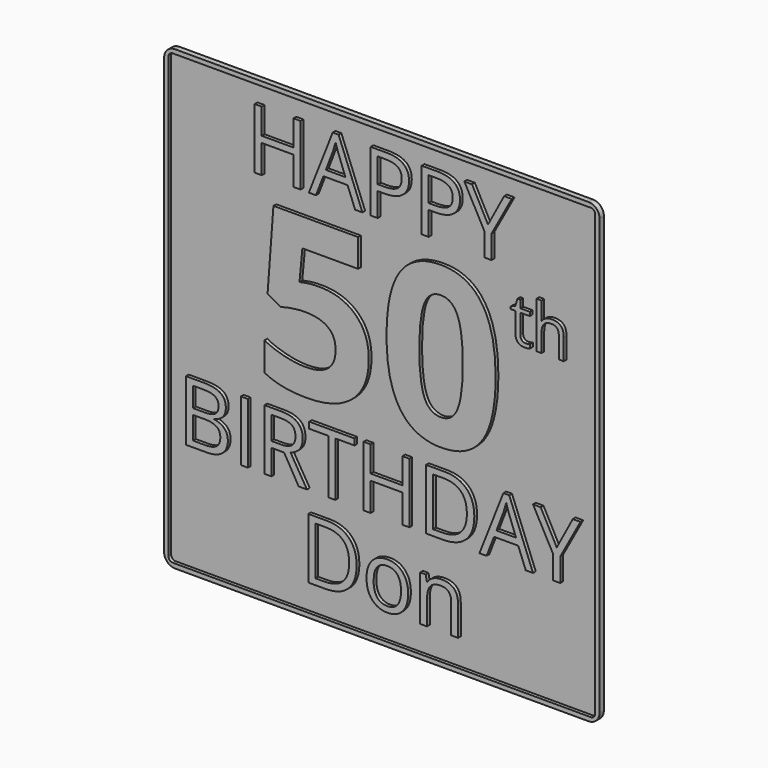
from build123d import *

# Parameters (mm, degrees)
F1_DEPTH       = 0.6
F2_TEXT_SIZE   = 24.6944444444
F2_TEXT_SIZE_2 = 63.7886434631
F2_TEXT_SIZE_3 = 17.7540454186
F3_DEPTH       = 1
F5_DEPTH       = 0.9906


# Not quite as in the source:
# - Text() gives the source's letters only with a copy of the font that has no kerning and outlines rounded to 1/6400 em; it was checked with that copy


with BuildPart() as f1:
    # F0 (on Front) → F1 (new body)
    with BuildSketch(Plane.XZ):
        with BuildLine():
            Line((123.825, 0), (3.175, 0))
            ThreePointArc((3.175, 0), (0.9299359697, -0.9299359697), (0, -3.175))
            Line((0, -3.175), (0, -130.175))
            ThreePointArc((0, -130.175), (0.9299359697, -132.4200640303), (3.175, -133.35))
            Line((3.175, -133.35), (123.825, -133.35))
            ThreePointArc((123.825, -133.35), (126.0700640303, -132.4200640303), (127, -130.175))
            Line((127, -130.175), (127, -3.175))
            ThreePointArc((127, -3.175), (126.0700640303, -0.9299359697), (123.825, 0))
        make_face()
    extrude(amount=F1_DEPTH)

    # F2 (on face) → F3 (join)
    with BuildSketch(Plane.XZ.offset(0.6)):
        with Locations((23.9946766493, -24.13)):
            Text('HAPPY', F2_TEXT_SIZE, font='Open Sans', text_align=(TextAlign.LEFT, TextAlign.BOTTOM))
        with Locations((3.9535915799, -100.5378232934)):
            Text('BIRTHDAY', F2_TEXT_SIZE, font='Open Sans', text_align=(TextAlign.LEFT, TextAlign.BOTTOM))
        with Locations((26.1587261352, -76.4078232934)):
            Text('50', F2_TEXT_SIZE_2, font='Open Sans', font_style=FontStyle.BOLD, text_align=(TextAlign.LEFT, TextAlign.BOTTOM))
        with Locations((100.8412738648, -43.2629127014)):
            Text('th', F2_TEXT_SIZE_3, font='Open Sans', text_align=(TextAlign.LEFT, TextAlign.BOTTOM))
        with Locations((39.6544270833, -124.3073880959)):
            Text('Don', F2_TEXT_SIZE, font='Open Sans', text_align=(TextAlign.LEFT, TextAlign.BOTTOM))
    extrude(amount=F3_DEPTH)

    # F4 (on face) → F5 (join)
    with BuildSketch(Plane.XZ.offset(0.6)):
        with BuildLine():
            Line((127, -130.175), (127, -3.175))
            ThreePointArc((127, -3.175), (126.0700640303, -0.9299359697), (123.825, 0))
            Line((123.825, 0), (3.175, 0))
            ThreePointArc((3.175, 0), (0.9299359697, -0.9299359697), (0, -3.175))
            Line((0, -3.175), (0, -130.175))
            ThreePointArc((0, -130.175), (0.9299359697, -132.4200640303), (3.175, -133.35))
            Line((3.175, -133.35), (123.825, -133.35))
            ThreePointArc((123.825, -133.35), (126.0700640303, -132.4200640303), (127, -130.175))
        make_face()
        with BuildLine():
            ThreePointArc((1.27, -2.54), (1.6419743879, -1.6419743879), (2.54, -1.27))
            Line((2.54, -1.27), (124.46, -1.27))
            ThreePointArc((124.46, -1.27), (125.3580256121, -1.6419743879), (125.73, -2.54))
            Line((125.73, -2.54), (125.73, -130.81))
            ThreePointArc((125.73, -130.81), (125.3580256121, -131.7080256121), (124.46, -132.08))
            Line((124.46, -132.08), (2.54, -132.08))
            ThreePointArc((2.54, -132.08), (1.6419743879, -131.7080256121), (1.27, -130.81))
            Line((1.27, -130.81), (1.27, -2.54))
        make_face(mode=Mode.SUBTRACT)
    extrude(amount=F5_DEPTH)


solid = f1.part
